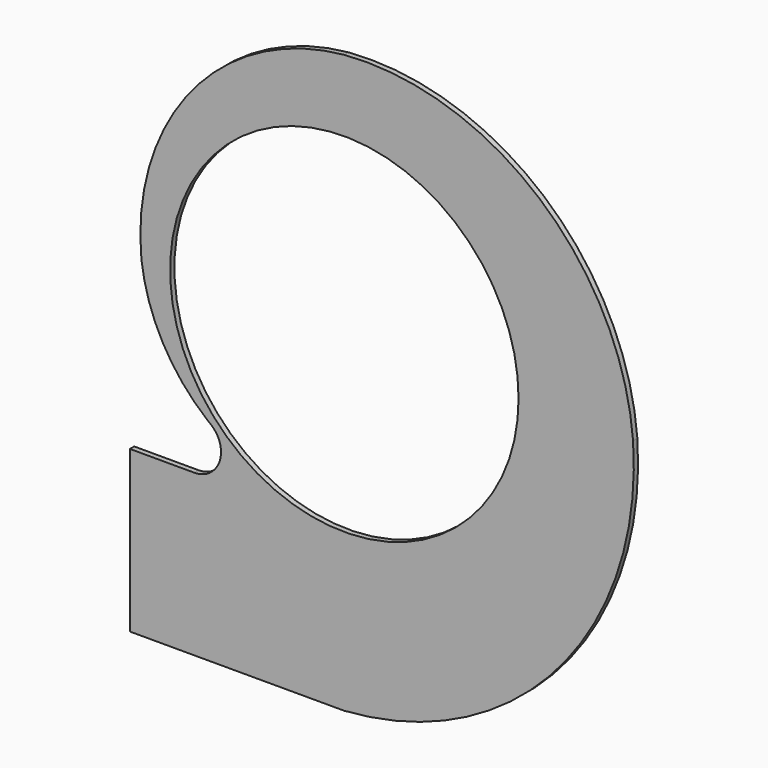
from build123d import *

# Parameters (mm, degrees)
F0_R     = 325
F1_DEPTH = 10


# Not quite as in the source:
# - a feature names something its author has since deleted; it is built from what else it names


with BuildPart() as f1:
    # F0 (on Front) → F1 (new body)
    with BuildSketch(Plane.XZ):
        with BuildLine():
            ThreePointArc((0, -618.6190456596), (397.429722157, -420.8611796621), (538.6190456596, 0))
            ThreePointArc((538.6190456596, 0), (364.2926371672, 340.8611796621), (0, 458.6190456596))
            ThreePointArc((0, 458.6190456596), (-284.2926371672, 307.7240946723), (-378.6190456596, 0))
            ThreePointArc((-378.6190456596, 0), (-338.9932719851, -123.9081492515), (-255.845498181, -223.9575325662))
            Line((-255.845498181, -223.9575325662), (-248.8807463186, -229.5026751274))
            ThreePointArc((-248.8807463186, -229.5026751274), (-232.823383589, -285.1142187928), (-280.0241173048, -318.6190456596))
            Line((-280.0241173048, -318.6190456596), (-400, -318.6190456596))
            Line((-400, -318.6190456596), (-400, -618.6190456596))
            Line((-400, -618.6190456596), (0, -618.6190456596))
        make_face()
        Circle(F0_R, mode=Mode.SUBTRACT)
    extrude(amount=F1_DEPTH)


solid = f1.part
